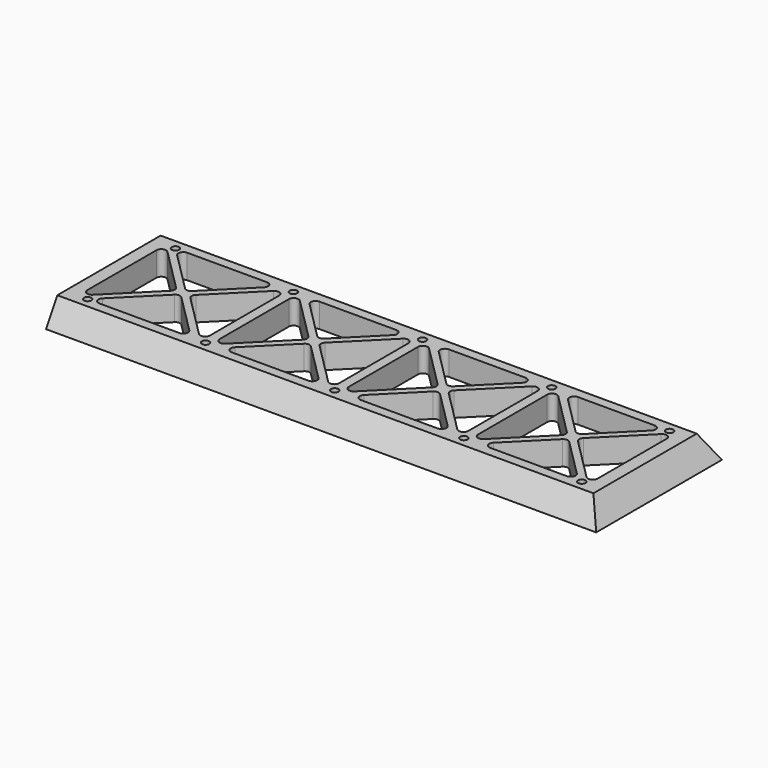
from build123d import *

# Parameters (mm, degrees)
F0_W      = 210.82
F0_H      = 50.8
F1_DEPTH  = 12.7
F3_DEPTH  = 10.16
F4_DEPTH  = 3.175
F6_DEPTH  = 210.82
F7_DEPTH  = 5.5118
F8_SIZE2  = 5.499251
F8_SIZE   = 9.52499
F9_R      = 1.4605
F10_DEPTH = 9.525


# Not quite as in the source:
# - a fillet or chamfer is up to 0.001 mm smaller than in the source, because OpenCascade refuses the exact size


with BuildPart() as f1:
    # F0 (on Top) → F1 (new body)
    with BuildSketch(Plane.XY):
        with Locations((105.41, 25.4)):
            Rectangle(F0_W, F0_H)
    extrude(amount=F1_DEPTH)

    # F2 (on face) → F3 (cut)
    with BuildSketch(Plane.XY.offset(12.7)):
        with BuildLine():
            ThreePointArc((8.3320384182, 43.7379615818), (6.2559880613, 44.1509136731), (5.08, 42.3909231637))
            Line((5.08, 42.3909231637), (5.08, 8.4090768363))
            ThreePointArc((5.08, 8.4090768363), (6.2559880613, 6.6490863269), (8.3320384182, 7.0620384182))
            Line((8.3320384182, 7.0620384182), (25.3229615818, 24.0529615818))
            ThreePointArc((25.3229615818, 24.0529615818), (25.8809231637, 25.4), (25.3229615818, 26.7470384182))
            Line((25.3229615818, 26.7470384182), (8.3320384182, 43.7379615818))
        make_face()
        with BuildLine():
            Line((50.0879615818, 43.7379615818), (33.0970384182, 26.7470384182))
            ThreePointArc((33.0970384182, 26.7470384182), (32.5390768363, 25.4), (33.0970384182, 24.0529615818))
            Line((33.0970384182, 24.0529615818), (50.0879615818, 7.0620384182))
            ThreePointArc((50.0879615818, 7.0620384182), (52.1640119387, 6.6490863269), (53.34, 8.4090768363))
            Line((53.34, 8.4090768363), (53.34, 42.3909231637))
            ThreePointArc((53.34, 42.3909231637), (52.1640119387, 44.1509136731), (50.0879615818, 43.7379615818))
        make_face()
        with BuildLine():
            ThreePointArc((60.4020384182, 43.7379615818), (58.3259880613, 44.1509136731), (57.15, 42.3909231637))
            Line((57.15, 42.3909231637), (57.15, 8.4090768363))
            ThreePointArc((57.15, 8.4090768363), (58.3259880613, 6.6490863269), (60.4020384182, 7.0620384182))
            Line((60.4020384182, 7.0620384182), (77.3929615818, 24.0529615818))
            ThreePointArc((77.3929615818, 24.0529615818), (77.9509231637, 25.4), (77.3929615818, 26.7470384182))
            Line((77.3929615818, 26.7470384182), (60.4020384182, 43.7379615818))
        make_face()
        with BuildLine():
            Line((104.14, 8.4090768363), (104.14, 42.3909231637))
            ThreePointArc((104.14, 42.3909231637), (102.9640119387, 44.1509136731), (100.8879615818, 43.7379615818))
            Line((100.8879615818, 43.7379615818), (83.8970384182, 26.7470384182))
            ThreePointArc((83.8970384182, 26.7470384182), (83.3390768363, 25.4), (83.8970384182, 24.0529615818))
            Line((83.8970384182, 24.0529615818), (100.8879615818, 7.0620384182))
            ThreePointArc((100.8879615818, 7.0620384182), (102.9640119387, 6.6490863269), (104.14, 8.4090768363))
        make_face()
        with BuildLine():
            ThreePointArc((111.2020384182, 43.7379615818), (109.1259880613, 44.1509136731), (107.95, 42.3909231637))
            Line((107.95, 42.3909231637), (107.95, 8.4090768363))
            ThreePointArc((107.95, 8.4090768363), (109.1259880613, 6.6490863269), (111.2020384182, 7.0620384182))
            Line((111.2020384182, 7.0620384182), (128.1929615818, 24.0529615818))
            ThreePointArc((128.1929615818, 24.0529615818), (128.7509231637, 25.4), (128.1929615818, 26.7470384182))
            Line((128.1929615818, 26.7470384182), (111.2020384182, 43.7379615818))
        make_face()
        with BuildLine():
            Line((154.94, 8.4090768363), (154.94, 42.3909231637))
            ThreePointArc((154.94, 42.3909231637), (153.7640119387, 44.1509136731), (151.6879615818, 43.7379615818))
            Line((151.6879615818, 43.7379615818), (134.6970384182, 26.7470384182))
            ThreePointArc((134.6970384182, 26.7470384182), (134.1390768363, 25.4), (134.6970384182, 24.0529615818))
            Line((134.6970384182, 24.0529615818), (151.6879615818, 7.0620384182))
            ThreePointArc((151.6879615818, 7.0620384182), (153.7640119387, 6.6490863269), (154.94, 8.4090768363))
        make_face()
        with BuildLine():
            ThreePointArc((162.0020384182, 43.7379615818), (159.9259880613, 44.1509136731), (158.75, 42.3909231637))
            Line((158.75, 42.3909231637), (158.75, 8.4090768363))
            ThreePointArc((158.75, 8.4090768363), (159.9259880613, 6.6490863269), (162.0020384182, 7.0620384182))
            Line((162.0020384182, 7.0620384182), (178.9929615818, 24.0529615818))
            ThreePointArc((178.9929615818, 24.0529615818), (179.5509231637, 25.4), (178.9929615818, 26.7470384182))
            Line((178.9929615818, 26.7470384182), (162.0020384182, 43.7379615818))
        make_face()
        with BuildLine():
            Line((205.74, 8.4090768363), (205.74, 42.3909231637))
            ThreePointArc((205.74, 42.3909231637), (204.5640119387, 44.1509136731), (202.4879615818, 43.7379615818))
            Line((202.4879615818, 43.7379615818), (185.4970384182, 26.7470384182))
            ThreePointArc((185.4970384182, 26.7470384182), (184.9390768363, 25.4), (185.4970384182, 24.0529615818))
            Line((185.4970384182, 24.0529615818), (202.4879615818, 7.0620384182))
            ThreePointArc((202.4879615818, 7.0620384182), (204.5640119387, 6.6490863269), (205.74, 8.4090768363))
        make_face()
        with BuildLine():
            Line((44.9309231637, 46.99), (13.4890768363, 46.99))
            ThreePointArc((13.4890768363, 46.99), (11.7290863269, 45.8140119387), (12.1420384182, 43.7379615818))
            Line((12.1420384182, 43.7379615818), (27.8629615818, 28.0170384182))
            ThreePointArc((27.8629615818, 28.0170384182), (29.21, 27.4590768363), (30.5570384182, 28.0170384182))
            Line((30.5570384182, 28.0170384182), (46.2779615818, 43.7379615818))
            ThreePointArc((46.2779615818, 43.7379615818), (46.6909136731, 45.8140119387), (44.9309231637, 46.99))
        make_face()
        with BuildLine():
            ThreePointArc((12.1420384182, 7.0620384182), (11.7290863269, 4.9859880613), (13.4890768363, 3.81))
            Line((13.4890768363, 3.81), (44.9309231637, 3.81))
            ThreePointArc((44.9309231637, 3.81), (46.6909136731, 4.9859880613), (46.2779615818, 7.0620384182))
            Line((46.2779615818, 7.0620384182), (30.5570384182, 22.7829615818))
            ThreePointArc((30.5570384182, 22.7829615818), (29.21, 23.3409231637), (27.8629615818, 22.7829615818))
            Line((27.8629615818, 22.7829615818), (12.1420384182, 7.0620384182))
        make_face()
        with BuildLine():
            Line((95.7309231637, 46.99), (65.5590768363, 46.99))
            ThreePointArc((65.5590768363, 46.99), (63.7990863269, 45.8140119387), (64.2120384182, 43.7379615818))
            Line((64.2120384182, 43.7379615818), (79.2979615818, 28.6520384182))
            ThreePointArc((79.2979615818, 28.6520384182), (80.645, 28.0940768363), (81.9920384182, 28.6520384182))
            Line((81.9920384182, 28.6520384182), (97.0779615818, 43.7379615818))
            ThreePointArc((97.0779615818, 43.7379615818), (97.4909136731, 45.8140119387), (95.7309231637, 46.99))
        make_face()
        with BuildLine():
            ThreePointArc((64.2120384182, 7.0620384182), (63.7990863269, 4.9859880613), (65.5590768363, 3.81))
            Line((65.5590768363, 3.81), (95.7309231637, 3.81))
            ThreePointArc((95.7309231637, 3.81), (97.4909136731, 4.9859880613), (97.0779615818, 7.0620384182))
            Line((97.0779615818, 7.0620384182), (81.9920384182, 22.1479615818))
            ThreePointArc((81.9920384182, 22.1479615818), (80.645, 22.7059231637), (79.2979615818, 22.1479615818))
            Line((79.2979615818, 22.1479615818), (64.2120384182, 7.0620384182))
        make_face()
        with BuildLine():
            Line((146.5309231637, 46.99), (116.3590768363, 46.99))
            ThreePointArc((116.3590768363, 46.99), (114.5990863269, 45.8140119387), (115.0120384182, 43.7379615818))
            Line((115.0120384182, 43.7379615818), (130.0979615818, 28.6520384182))
            ThreePointArc((130.0979615818, 28.6520384182), (131.445, 28.0940768363), (132.7920384182, 28.6520384182))
            Line((132.7920384182, 28.6520384182), (147.8779615818, 43.7379615818))
            ThreePointArc((147.8779615818, 43.7379615818), (148.2909136731, 45.8140119387), (146.5309231637, 46.99))
        make_face()
        with BuildLine():
            ThreePointArc((115.0120384182, 7.0620384182), (114.5990863269, 4.9859880613), (116.3590768363, 3.81))
            Line((116.3590768363, 3.81), (146.5309231637, 3.81))
            ThreePointArc((146.5309231637, 3.81), (148.2909136731, 4.9859880613), (147.8779615818, 7.0620384182))
            Line((147.8779615818, 7.0620384182), (132.7920384182, 22.1479615818))
            ThreePointArc((132.7920384182, 22.1479615818), (131.445, 22.7059231637), (130.0979615818, 22.1479615818))
            Line((130.0979615818, 22.1479615818), (115.0120384182, 7.0620384182))
        make_face()
        with BuildLine():
            Line((197.3309231637, 46.99), (167.1590768363, 46.99))
            ThreePointArc((167.1590768363, 46.99), (165.3990863269, 45.8140119387), (165.8120384182, 43.7379615818))
            Line((165.8120384182, 43.7379615818), (180.8979615818, 28.6520384182))
            ThreePointArc((180.8979615818, 28.6520384182), (182.245, 28.0940768363), (183.5920384182, 28.6520384182))
            Line((183.5920384182, 28.6520384182), (198.6779615818, 43.7379615818))
            ThreePointArc((198.6779615818, 43.7379615818), (199.0909136731, 45.8140119387), (197.3309231637, 46.99))
        make_face()
        with BuildLine():
            ThreePointArc((165.8120384182, 7.0620384182), (165.3990863269, 4.9859880613), (167.1590768363, 3.81))
            Line((167.1590768363, 3.81), (197.3309231637, 3.81))
            ThreePointArc((197.3309231637, 3.81), (199.0909136731, 4.9859880613), (198.6779615818, 7.0620384182))
            Line((198.6779615818, 7.0620384182), (183.5920384182, 22.1479615818))
            ThreePointArc((183.5920384182, 22.1479615818), (182.245, 22.7059231637), (180.8979615818, 22.1479615818))
            Line((180.8979615818, 22.1479615818), (165.8120384182, 7.0620384182))
        make_face()
    extrude(amount=-F3_DEPTH, mode=Mode.SUBTRACT)

    # F4 (cut): a face of the model
    f4_faces = [f1.faces().sort_by_distance(p)[0] for p in [
        (105.41, 25.4, 0),
    ]]
    extrude(f4_faces, amount=-F4_DEPTH, mode=Mode.SUBTRACT)

    # F5 (on face) → F6 (join)
    with BuildSketch(Plane(origin=(0, 0, 0), x_dir=(0, -1, 0), z_dir=(-1, 0, 0))):
        Polygon((-56.299261314, 3.175), (-50.8, 3.175), (-50.8, 12.7), align=None)
        Polygon((0, 12.7), (0, 3.175), (5.499261314, 3.175), align=None)
    extrude(amount=-F6_DEPTH)

    # F7 (add): a face of the model
    f7_faces = [f1.faces().sort_by_distance(p)[0] for p in [
        (210.82, 25.4, 7.7824344249),
    ]]
    extrude(f7_faces, amount=F7_DEPTH)

    # F8 (size 9.525 and 5.499261314 in the source; OpenCascade refuses exactly that, so slightly less here)
    f8_edges = [f1.edges().sort_by_distance(p)[0] for p in [
        (216.3318, 25.4, 12.7),
    ]]
    f8_side = f1.faces().sort_by_distance((216.3318, 25.4, 7.782434))[0]
    chamfer(f8_edges, length=F8_SIZE, length2=F8_SIZE2, reference=f8_side)

    # F9 (on face) → F10 (cut)
    with BuildSketch(Plane.XY.offset(12.7)):
        with Locations((8.89, 46.99)):
            Circle(F9_R)
        with Locations((8.89, 3.81)):
            Circle(F9_R)
        with Locations((55.245, 46.99)):
            Circle(F9_R)
        with Locations((55.245, 3.81)):
            Circle(F9_R)
        with Locations((106.045, 46.99)):
            Circle(F9_R)
        with Locations((106.045, 3.81)):
            Circle(F9_R)
        with Locations((156.845, 46.99)):
            Circle(F9_R)
        with Locations((156.845, 3.81)):
            Circle(F9_R)
        with Locations((203.2, 46.99)):
            Circle(F9_R)
        with Locations((203.2, 3.81)):
            Circle(F9_R)
    extrude(amount=-F10_DEPTH, mode=Mode.SUBTRACT)


solid = f1.part
